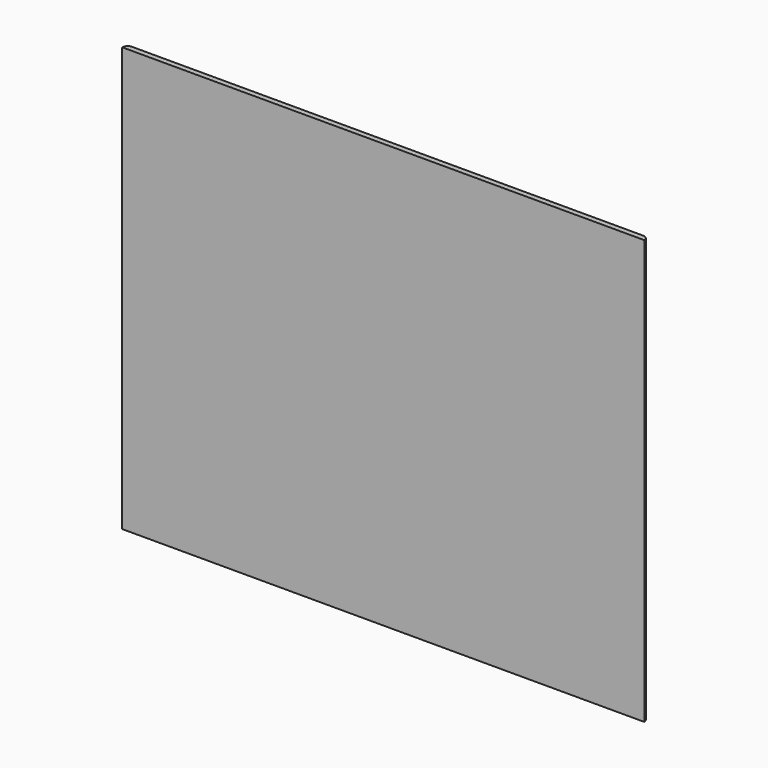
from build123d import *

# Parameters (mm, degrees)
F0_W     = 1219.2
F0_H     = 990.6
F1_DEPTH = 12.7
F2_R     = 12.69999


# Not quite as in the source:
# - a fillet or chamfer is up to 0.001 mm smaller than in the source, because OpenCascade refuses the exact size


with BuildPart() as f1:
    # F0 (on Front) → F1 (new body)
    with BuildSketch(Plane.XZ):
        Rectangle(F0_W, F0_H)
    extrude(amount=F1_DEPTH)

    # F2 (radius 12.7 in the source; OpenCascade refuses exactly that, so slightly less here)
    f2_edges = [f1.edges().sort_by_distance(p)[0] for p in [
        (609.6, 0, 0),
        (-609.6, 0, 0),
    ]]
    fillet(f2_edges, radius=F2_R)


solid = f1.part
